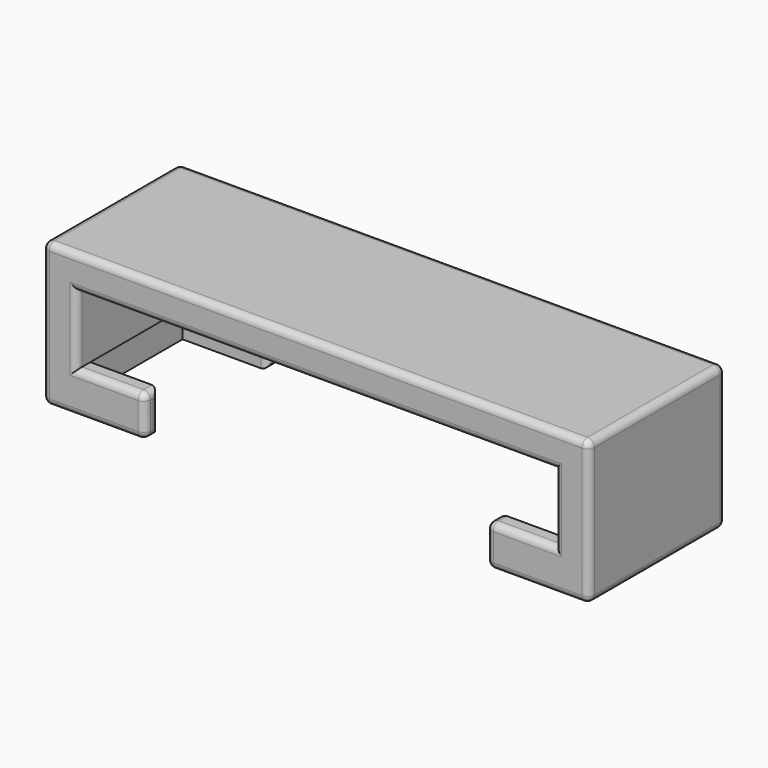
from build123d import *

# Parameters (mm, degrees)
F1_DEPTH    = 25
F2_T        = 2.5
F2_T3_DEPTH = 30
F3_R        = 1


# Not quite as in the source:
# - a shell that OpenCascade refuses in one call is made with other operations: the cavity is built on its own and cut out


with BuildPart() as f1:
    # F0 (on Front) → F1 (new body)
    with BuildSketch(Plane.XZ):
        Polygon((-48.0838582665, 23.83404883), (-48.0838582665, 33.83404883), (21.9161417335, 33.83404883), (21.9161417335, 23.83404883), (11.9161417335, 23.83404883), (11.9161417335, 17.83404883), (21.9161417335, 17.83404883), (26.9161417335, 17.83404883), (26.9161417335, 38.83404883), (-53.0838582665, 38.83404883), (-53.0838582665, 17.83404883), (-48.0838582665, 17.83404883), (-38.0838582665, 17.83404883), (-38.0838582665, 23.83404883), align=None)
    extrude(amount=F1_DEPTH)

    # F2: shell of thickness 2.5, made by hand


with BuildPart() as f2_core1:
    # F2_t2: copy of F1
    add(f1.part)

    # the walls: a layer under each face that stays
    f2_faces = [f2_core1.faces().sort_by_distance(p)[0] for p in [
        (21.9161417335, -12.5, 28.83404883),
        (-39.7505249331, -25, 21.33404883),
        (-48.0838582665, -12.5, 28.83404883),
        (-53.0838582665, -12.5, 28.33404883),
        (-13.0838582665, -12.5, 38.83404883),
        (26.9161417335, -12.5, 28.33404883),
        (-39.7505249331, 0, 21.33404883),
        (-13.0838582665, -12.5, 33.83404883),
    ]]
    thicken(f2_faces, amount=-F2_T, mode=Mode.SUBTRACT)

    # F2_s4 → F2_t3 (cut)
    with BuildSketch(Plane.XZ.offset(-2.5)):
        Polygon((21.8911417335, 33.80904883), (24.4161417335, 33.83404883), (24.4161417335, 36.33404883), (21.9161417335, 36.33404883), align=None)
        Polygon((-48.0588582665, 33.80904883), (-50.5838582665, 33.83404883), (-50.5838582665, 36.33404883), (-48.0838582665, 36.33404883), align=None)
    extrude(amount=F2_T3_DEPTH, mode=Mode.SUBTRACT)


with BuildPart() as f1_1:
    add(f1.part)

    # what is left inside the walls is the cavity
    f2_cavity = [f2_core1.part.solids().sort_by_distance(p)[0] for p in [
        (18.166142, -15.833333, 23.809049),
        (-44.333858, -15.833333, 23.809049),
    ]]
    add(f2_cavity, mode=Mode.SUBTRACT)

    # F3
    f3_edges = [f1_1.edges().sort_by_distance(p)[0] for p in [
        (-38.083858, 0, 20.834049),
        (-38.083858, -1.25, 23.834049),
        (-38.083858, -2.5, 20.834049),
        (-38.083858, -1.25, 17.834049),
        (-38.083858, -22.5, 20.834049),
        (-38.083858, -23.75, 23.834049),
        (-38.083858, -25, 20.834049),
        (-38.083858, -23.75, 17.834049),
        (11.916142, 0, 20.834049),
        (11.916142, -1.25, 17.834049),
        (11.916142, -2.5, 20.834049),
        (11.916142, -1.25, 23.834049),
        (11.916142, -22.5, 20.834049),
        (11.916142, -23.75, 17.834049),
        (11.916142, -25, 20.834049),
        (11.916142, -23.75, 23.834049),
        (21.916142, 0, 28.834049),
        (16.916142, 0, 23.834049),
        (19.416142, 0, 17.834049),
        (26.916142, 0, 28.334049),
        (-13.083858, 0, 38.834049),
        (-53.083858, 0, 28.334049),
        (-45.583858, 0, 17.834049),
        (-43.083858, 0, 23.834049),
        (-48.083858, 0, 28.834049),
        (-13.083858, 0, 33.834049),
        (26.916142, -12.5, 17.834049),
        (26.916142, -12.5, 38.834049),
        (26.916142, -25, 28.334049),
        (21.916142, -25, 28.834049),
        (16.916142, -25, 23.834049),
        (19.416142, -25, 17.834049),
        (-13.083858, -25, 38.834049),
        (-53.083858, -25, 28.334049),
        (-45.583858, -25, 17.834049),
        (-43.083858, -25, 23.834049),
        (-48.083858, -25, 28.834049),
        (-13.083858, -25, 33.834049),
        (-53.083858, -12.5, 38.834049),
        (-53.083858, -12.5, 17.834049),
    ]]
    fillet(f3_edges, radius=F3_R)


solid = f1_1.part
